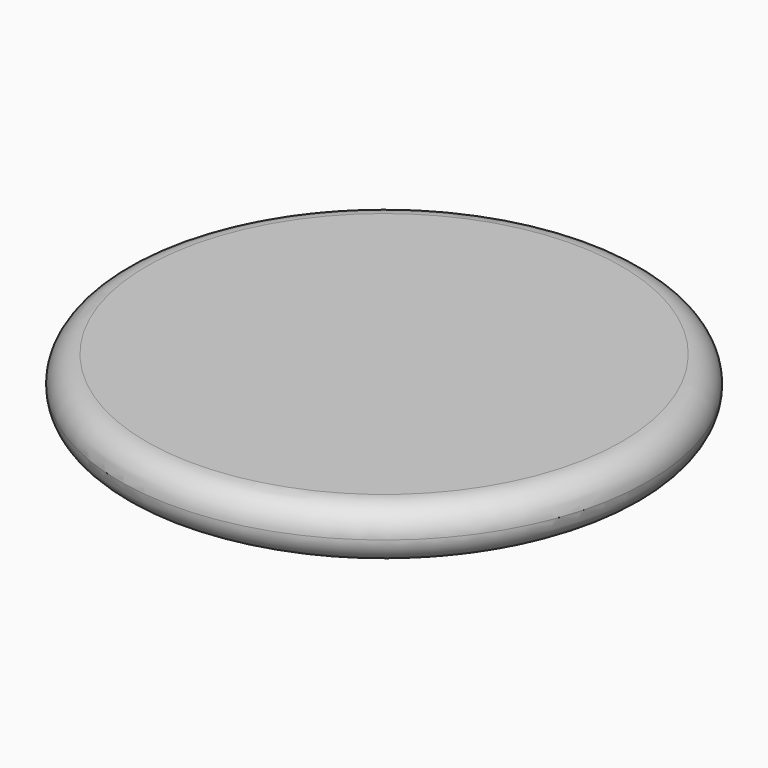
from build123d import *

# Parameters (mm, degrees)
F0_R     = 50
F1_DEPTH = 10
F2_R     = 5
F3_R     = 4.99999


# Not quite as in the source:
# - a fillet or chamfer is up to 0.001 mm smaller than in the source, because OpenCascade refuses the exact size


with BuildPart() as f1:
    # F0 (on Top) → F1 (new body)
    with BuildSketch(Plane.XY):
        Circle(F0_R)
    extrude(amount=F1_DEPTH)

    # F2
    f2_edges = [f1.edges().sort_by_distance(p)[0] for p in [
        (-50, 0, 10),
    ]]
    fillet(f2_edges, radius=F2_R)

    # F3 (radius 5 in the source; OpenCascade refuses exactly that, so slightly less here)
    f3_edges = [f1.edges().sort_by_distance(p)[0] for p in [
        (-50, 0, 0),
    ]]
    fillet(f3_edges, radius=F3_R)


solid = f1.part
